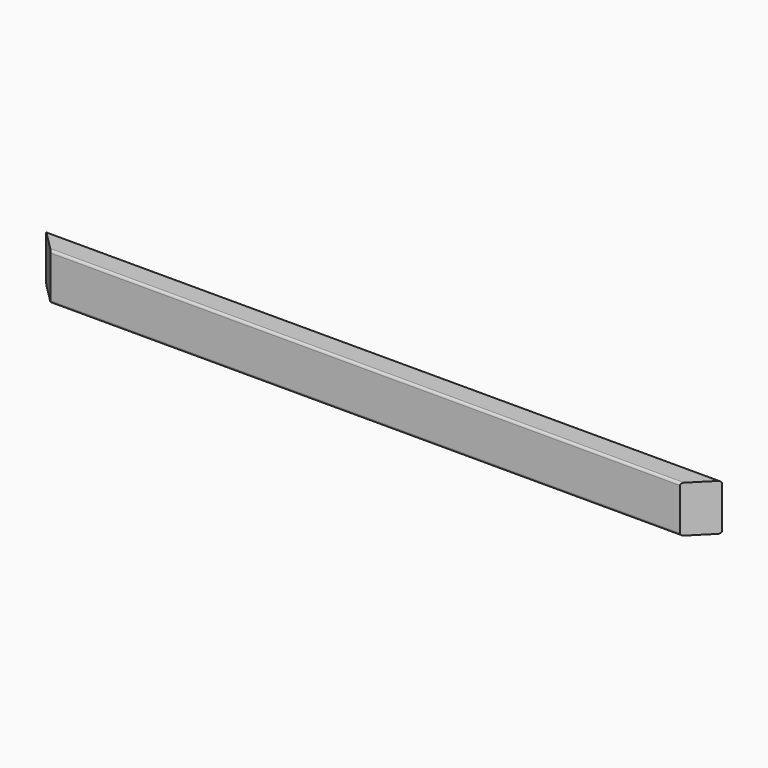
from build123d import *

# Parameters (mm, degrees)
F0_W     = 1450
F0_H     = 100
F4_DEPTH = 50
F1_SIZE  = 49.99999
F2_SIZE  = 49.99999
F3_R     = 5


# Not quite as in the source:
# - a fillet or chamfer is up to 0.001 mm smaller than in the source, because OpenCascade refuses the exact size


with BuildPart() as f4:
    # F0 (on Front) → F4 (new body)
    with BuildSketch(Plane.XZ):
        with Locations((74.6626051481, 50)):
            Rectangle(F0_W, F0_H)
    extrude(amount=F4_DEPTH)

    # F1 (size 50 in the source; OpenCascade refuses exactly that, so slightly less here)
    f1_edges = [f4.edges().sort_by_distance(p)[0] for p in [
        (799.662605, -50, 50),
    ]]
    chamfer(f1_edges, length=F1_SIZE)

    # F2 (size 50 in the source; OpenCascade refuses exactly that, so slightly less here)
    f2_edges = [f4.edges().sort_by_distance(p)[0] for p in [
        (-650.337395, -50, 50),
    ]]
    chamfer(f2_edges, length=F2_SIZE)

    # F3
    f3_edges = [f4.edges().sort_by_distance(p)[0] for p in [
        (74.662605, -50, 100),
        (74.662605, -50, 0),
        (74.662605, 0, 100),
        (74.662605, 0, 0),
    ]]
    fillet(f3_edges, radius=F3_R)


solid = f4.part
